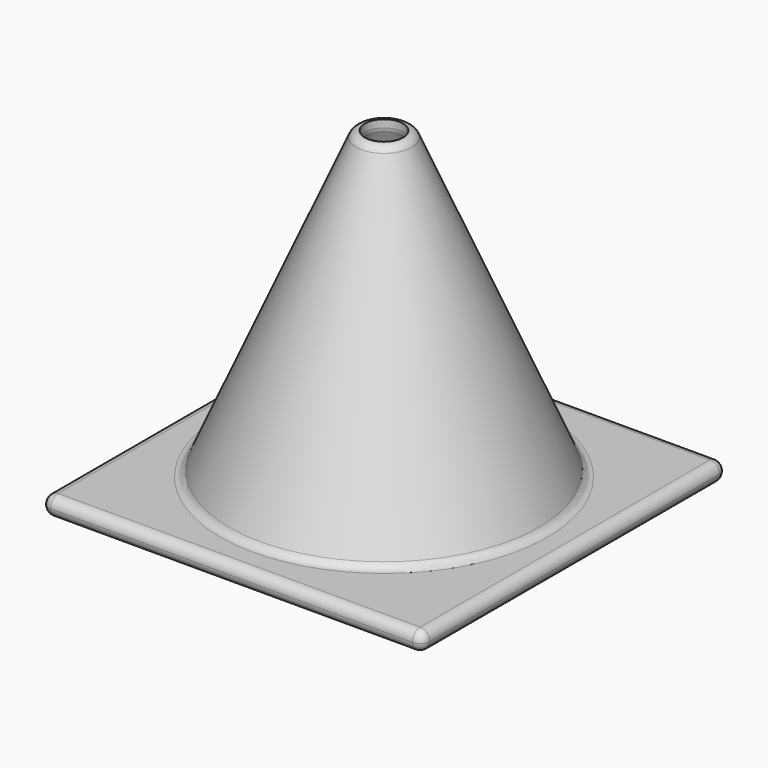
from build123d import *

# Parameters (mm, degrees)
F2_W     = 200
F2_H     = 200
F2_R     = 82.6159275748
F2_R_2   = 75.2160474693
F3_DEPTH = 10
F4_R     = 4.99999


# Not quite as in the source:
# - a fillet or chamfer is up to 0.001 mm smaller than in the source, because OpenCascade refuses the exact size


with BuildPart() as f1:
    # F0 (on Front) → F1 (revolve)
    with BuildSketch(Plane.XZ):
        Polygon((-75, -75), (-10, 75), (-10, 80), (-13.2825942414, 80), (-82.6159275748, -80), (-75, -80), align=None)
    revolve(axis=Axis((0, 0, 2.9210224748), (0, 0, 1)))

    # F2 (on face) → F3 (join)
    with BuildSketch(Plane(origin=(0, 0, -80), x_dir=(1, 0, 0), z_dir=(0, 0, -1))):
        Rectangle(F2_W, F2_H)
        Circle(F2_R, mode=Mode.SUBTRACT)
        Circle(F2_R)
        Circle(F2_R_2, mode=Mode.SUBTRACT)
    extrude(amount=F3_DEPTH)

    # F4 (radius 5 in the source; OpenCascade refuses exactly that, so slightly less here)
    f4_edges = [f1.edges().sort_by_distance(p)[0] for p in [
        (-100, 100, -85),
        (100, 100, -85),
        (100, -100, -85),
        (-75.216047, 0, -90),
        (75, 0, -75),
        (-100, -100, -85),
        (0, 100, -90),
        (100, 0, -90),
        (0, -100, -90),
        (-100, 0, -90),
        (0, 100, -80),
        (-100, 0, -80),
        (100, 0, -80),
        (0, -100, -80),
        (82.615928, 0, -80),
        (13.282594, 0, 80),
        (10, 0, 75),
    ]]
    fillet(f4_edges, radius=F4_R)


solid = f1.part
